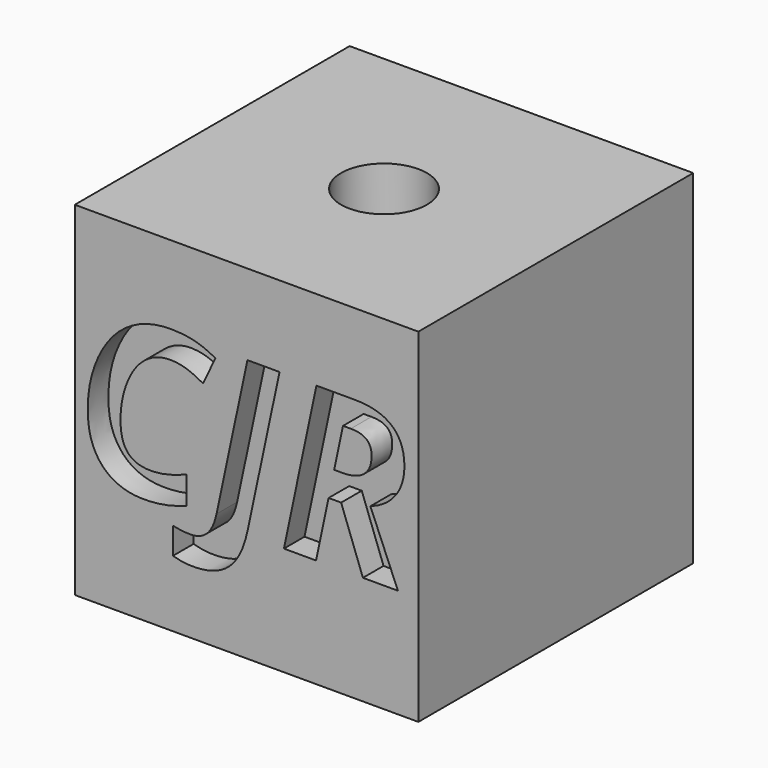
from build123d import *

# Parameters (mm, degrees)
F0_W         = 40
F0_H         = 40
F1_DEPTH     = 20
F2_TEXT_SIZE = 25.1276010993
F3_DEPTH     = 3
F4_R         = 5
F5_DEPTH     = 10
F6_R         = 5
F7_DEPTH     = 10
F8_R         = 5
F9_DEPTH     = 10


# Not quite as in the source:
# - Text() gives the source's letters only with a copy of the font that has no kerning and outlines rounded to 1/6400 em; it was checked with that copy


with BuildPart() as f1:
    # F0 (on Front) → F1 (new body, symmetric)
    with BuildSketch(Plane.XZ):
        Rectangle(F0_W, F0_H)
    extrude(amount=F1_DEPTH, both=True)

    # F2 (on face) → F3 (cut)
    with BuildSketch(Plane.XZ.offset(20)):
        with Locations((-20, -7.3272744165)):
            Text('CJR', F2_TEXT_SIZE, font='Open Sans', font_style=FontStyle.BOLDITALIC, text_align=(TextAlign.LEFT, TextAlign.BOTTOM))
    extrude(amount=-F3_DEPTH, mode=Mode.SUBTRACT)

    # F4 (on face) → F5 (cut)
    with BuildSketch(Plane(origin=(-20, 0, 0), x_dir=(0, -1, 0), z_dir=(-1, 0, 0))):
        Circle(F4_R)
    extrude(amount=-F5_DEPTH, mode=Mode.SUBTRACT)

    # F6 (on face) → F7 (cut)
    with BuildSketch(Plane(origin=(0, 0, -20), x_dir=(1, 0, 0), z_dir=(0, 0, -1))):
        Circle(F6_R)
    extrude(amount=-F7_DEPTH, mode=Mode.SUBTRACT)

    # F8 (on face) → F9 (cut)
    with BuildSketch(Plane.XY.offset(20)):
        Circle(F8_R)
    extrude(amount=-F9_DEPTH, mode=Mode.SUBTRACT)


solid = f1.part
